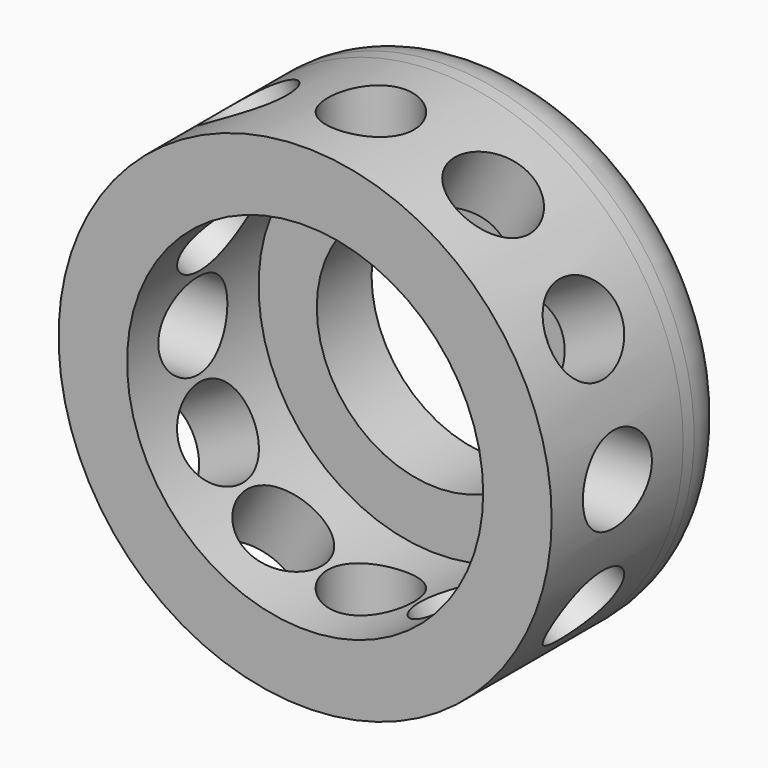
from build123d import *

# Parameters (mm, degrees)
F0_R            = 22.86
F0_R_2          = 16.51
F1_DEPTH        = 7.62
F2_R            = 4
F3_DEPTH        = 77.216
F3_COPIES_COUNT = 12
F4_R            = 22.86
F5_DEPTH        = 6.35
F6_R            = 11.1125
F7_DEPTH        = 25.4
F8_R            = 5.08


# Not quite as in the source:
# - a pattern or mirror of a feature is missing from the dataset's text; its kind, count and spacing are read off the source's solid


with BuildPart() as f1:
    # F0 (on Front) → F1 (new body, symmetric)
    with BuildSketch(Plane.XZ):
        Circle(F0_R)
        Circle(F0_R_2, mode=Mode.SUBTRACT)
    extrude(amount=F1_DEPTH, both=True)

    # F2 (on Top) → F3 (cut)
    with BuildSketch(Plane.XY):
        Circle(F2_R)
    f3 = extrude(amount=F3_DEPTH, mode=Mode.SUBTRACT)

    # F3_copies: F3 ×12 about axis
    f3_copies_axis = Axis((0, 0, 0), (0, 1, 0))
    for i in range(1, F3_COPIES_COUNT):
        add(f3.rotate(f3_copies_axis, i * 360 / F3_COPIES_COUNT), mode=Mode.SUBTRACT)

    # F4 (on face) → F5 (join)
    with BuildSketch(Plane(origin=(0, 7.62, 0), x_dir=(-1, 0, 0), z_dir=(0, 1, 0))):
        Circle(F4_R)
    extrude(amount=F5_DEPTH)

    # F6 (on face) → F7 (cut)
    with BuildSketch(Plane(origin=(0, 13.97, 0), x_dir=(-1, 0, 0), z_dir=(0, 1, 0))):
        Circle(F6_R)
    extrude(amount=-F7_DEPTH, mode=Mode.SUBTRACT)

    # F8
    f8_edges = [f1.edges().sort_by_distance(p)[0] for p in [
        (22.86, 13.97, 0),
    ]]
    fillet(f8_edges, radius=F8_R)


solid = f1.part
